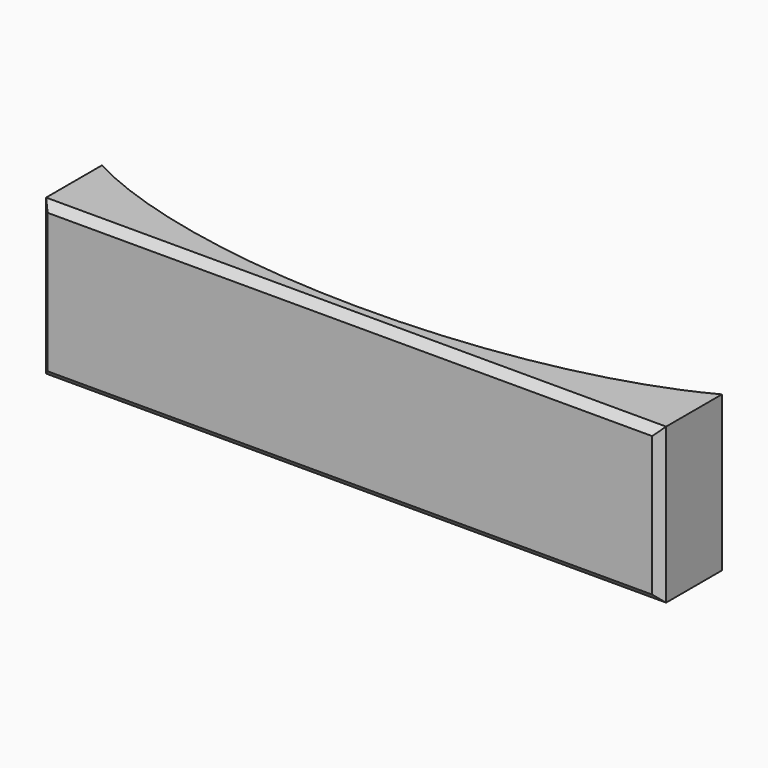
from build123d import *

# Parameters (mm, degrees)
F1_DEPTH = 20
F2_SIZE  = 1


with BuildPart() as f1:
    # F0 (on Top) → F1 (new body)
    with BuildSketch(Plane.XY):
        with BuildLine():
            add(Edge.make_bspline(
                [(-40, -12), (0, -33.3333333333), (40, -12)],
                knots=[3.7850937624, 3.7850937624, 3.7850937624, 5.6396841984, 5.6396841984, 5.6396841984], degree=2, weights=[1, 0.6, 1]))
            Line((-40, -12), (-40, -22))
            Line((-40, -22), (40, -22))
            Line((40, -22), (40, -12))
        make_face()
    extrude(amount=F1_DEPTH)

    # F2
    f2_edges = [f1.edges().sort_by_distance(p)[0] for p in [
        (-40, -22, 10),
        (0, -22, 20),
        (0, -22, 0),
        (40, -22, 10),
    ]]
    chamfer(f2_edges, length=F2_SIZE)


solid = f1.part
